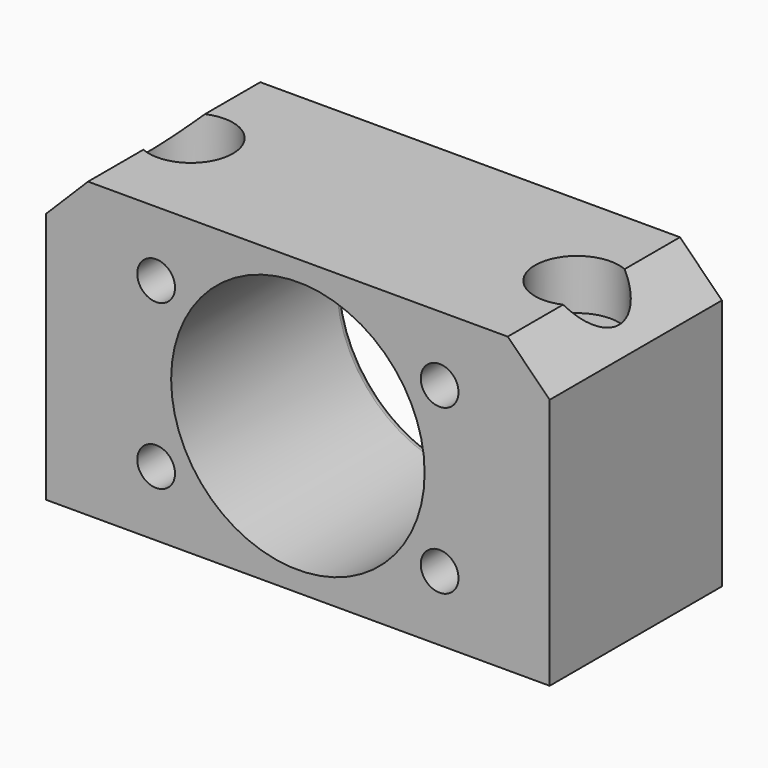
from build123d import *

# Parameters (mm, degrees)
F0_W           = 60
F0_H           = 35
F0_R           = 2.25
F0_R_2         = 15.1
F1_DEPTH       = 25.65
F3_D           = 5.5
F3_DEPTH       = 35
F3_CBORE_D     = 10
F3_CBORE_DEPTH = 6
F3_TIP         = 1.6523667023
F4_T1_DEPTH    = 51.3668298797
F5_R           = 1


# Not quite as in the source:
# - a fillet or chamfer that OpenCascade refuses, or shapes differently, is made with other operations: its cross-section is extruded or revolved along the edge and cut away or added


with BuildPart() as f1:
    # F0 (on Front) → F1 (new body)
    with BuildSketch(Plane.XZ):
        Rectangle(F0_W, F0_H)
        with Locations((-16.8874953738, -9.75)):
            Circle(F0_R, mode=Mode.SUBTRACT)
        with Locations((16.8874953738, -9.75)):
            Circle(F0_R, mode=Mode.SUBTRACT)
        with Locations((-16.8874953738, 9.75)):
            Circle(F0_R, mode=Mode.SUBTRACT)
        Circle(F0_R_2, mode=Mode.SUBTRACT)
        with Locations((16.8874953738, 9.75)):
            Circle(F0_R, mode=Mode.SUBTRACT)
    extrude(amount=-F1_DEPTH)

    # F3
    with Locations(Plane.XY.offset(17.5)):
        with Locations((-23, 12.825), (23, 12.825)):
            CounterBoreHole(F3_D / 2, F3_CBORE_D / 2, F3_CBORE_DEPTH, depth=F3_DEPTH)
            with Locations((0, 0, -(F3_DEPTH + F3_TIP / 2))):  # 118° drill point
                Cone(0, F3_D / 2, F3_TIP, mode=Mode.SUBTRACT)

    # F4: chamfer of 5 on 2 edges, made by hand

    # F4_s2 → F4_t1 (cut)
    with BuildSketch(Plane.XZ.offset(-38.5084149398)):
        Polygon((25, 17.5), (30, 12.5), (30, 17.5), align=None)
        Polygon((-30, 12.5), (-25, 17.5), (-30, 17.5), align=None)
    extrude(amount=F4_T1_DEPTH, mode=Mode.SUBTRACT)

    # F5
    f5_edges = [f1.edges().sort_by_distance(p)[0] for p in [
        (-15.1, 25.65, 0),
    ]]
    fillet(f5_edges, radius=F5_R)


solid = f1.part
